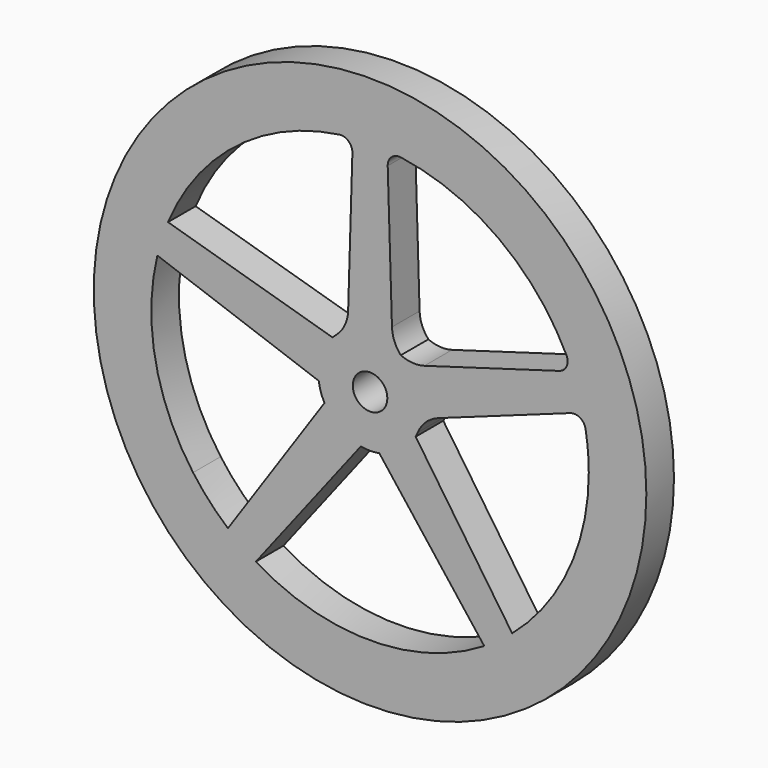
from build123d import *

# Parameters (mm, degrees)
F0_R        = 24
F0_R_2      = 1.5
F1_DEPTH    = 3
F2_COUNT    = 5
F3_T1_DEPTH = 3
F4_R        = 1


# Not quite as in the source:
# - a fillet or chamfer that OpenCascade refuses, or shapes differently, is made with other operations: its cross-section is extruded or revolved along the edge and cut away or added


with BuildPart() as f1:
    # F0 (on Front) → F1 (new body)
    with BuildSketch(Plane.XZ):
        Circle(F0_R)
        with BuildLine():
            ThreePointArc((-1.4988309156, 18.9407894737), (0, 19), (1.4988309156, 18.9407894737))
            ThreePointArc((1.4988309156, 18.9407894737), (13.9548878067, 12.8942276349), (19, 0))
            ThreePointArc((19, 0), (-12.8942276349, -13.9548878067), (-1.4988309156, 18.9407894737))
        make_face(mode=Mode.SUBTRACT)
        with BuildLine():
            ThreePointArc((-1.9499920861, 4.0555555556), (-2.3953116303, -3.8095251927), (4.5, 0))
            ThreePointArc((4.5, 0), (3.8095251927, 2.3953116303), (1.9499920861, 4.0555555556))
            ThreePointArc((1.9499920861, 4.0555555556), (0, 4.5), (-1.9499920861, 4.0555555556))
        make_face()
        Circle(F0_R_2, mode=Mode.SUBTRACT)
        with BuildLine():
            ThreePointArc((-1.9499920861, 4.0555555556), (0, 4.5), (1.9499920861, 4.0555555556))
            Line((1.9499920861, 4.0555555556), (1.4988309156, 18.9407894737))
            ThreePointArc((1.4988309156, 18.9407894737), (0, 19), (-1.4988309156, 18.9407894737))
            Line((-1.4988309156, 18.9407894737), (-1.9499920861, 4.0555555556))
        make_face()
    extrude(amount=F1_DEPTH)

    # F2: F1 ×5 about axis
    f2_axis = Axis((0, 0, 0), (0, 1, 0))


with BuildPart() as f1_1:
    add(f1.part)
    for i in range(1, F2_COUNT):
        add(f1.part.rotate(f2_axis, i * 360 / F2_COUNT))

    # F3: fillet of radius 3 on 4 edges, made by hand

    # F3_s2 → F3_t1 (join)
    with BuildSketch(Plane.XZ):
        with BuildLine():
            ThreePointArc((-2.9413516087, 3.4056498225), (-2.1935950838, 4.3864419946), (-1.903629714, 5.5851968442))
            Line((-1.903629714, 5.5851968442), (-1.9499920861, 4.0555555556))
            ThreePointArc((-1.9499920861, 4.0555555556), (-2.467165408, 3.7633887454), (-2.9413516087, 3.4056498225))
        make_face()
        with BuildLine():
            ThreePointArc((2.3300378224, 3.8497952863), (3.4938960826, 3.4417180197), (4.7235839209, 3.5363801859))
            Line((4.7235839209, 3.5363801859), (3.2544818448, 3.1077882685))
            ThreePointArc((3.2544818448, 3.1077882685), (2.8167993507, 3.5093648169), (2.3300378224, 3.8497952863))
        make_face()
        with BuildLine():
            ThreePointArc((1.903629714, 5.5851968442), (2.1935950838, 4.3864419946), (2.9413516087, 3.4056498225))
            ThreePointArc((2.9413516087, 3.4056498225), (2.467165408, 3.7633887454), (1.9499920861, 4.0555555556))
            Line((1.9499920861, 4.0555555556), (1.903629714, 5.5851968442))
        make_face()
        with BuildLine():
            ThreePointArc((5.9000917861, -0.0845387023), (4.8496124019, -0.7307477774), (4.1478930895, -1.7449879421))
            ThreePointArc((4.1478930895, -1.7449879421), (4.3415914287, -1.1834626593), (4.4596432318, -0.6013170919))
            Line((4.4596432318, -0.6013170919), (5.9000917861, -0.0845387023))
        make_face()
    extrude(amount=F3_T1_DEPTH)

    # F4
    f4_edges = [f1_1.edges().sort_by_distance(p)[0] for p in [
        (-1.498831, -1.5, 18.940789),
        (17.550597, -1.5, 7.278499),
        (18.476925, -1.5, 4.427553),
        (1.498831, -1.5, 18.940789),
    ]]
    fillet(f4_edges, radius=F4_R)


solid = f1_1.part
